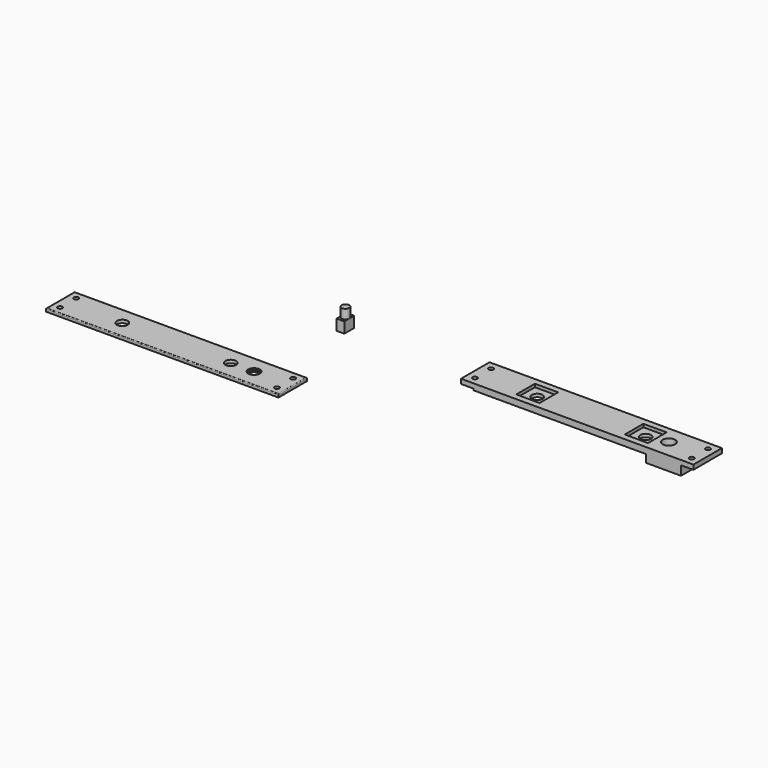
from build123d import *

# Parameters (mm, degrees)
F1_W      = 5
F1_H      = 8
F2_DEPTH  = 7
F4_DEPTH  = 6
F0_W      = 150
F0_H      = 23
F0_R      = 1.5
F0_R_2    = 3.5
F0_R_3    = 4
F5_DEPTH  = 4
F6_W      = 150
F6_H      = 23
F6_R      = 1.5
F6_R_2    = 3.5
F6_R_3    = 3.1
F7_DEPTH  = 2
F8_R      = 3.75
F9_DEPTH  = 1
F10_W     = 8
F10_H     = 1
F11_DEPTH = 30
F12_W     = 15
F12_H     = 15
F12_R     = 3.5
F13_DEPTH = 2
F14_R     = 4
F15_DEPTH = 3
F17_R     = 0.5
F16_W     = 22.5
F16_H     = 23
F16_R     = 4
F18_DEPTH = 5
F19_W     = 3
F19_H     = 7.4161984871
F20_DEPTH = 2


with BuildPart() as f2:
    # F1 (on Top) → F2 (new body)
    with BuildSketch(Plane.XY):
        with Locations((-158.8816171885, 0.1063133087)):
            Rectangle(F1_W, F1_H)
    extrude(amount=F2_DEPTH)

    # F3 (on face) → F4 (join)
    with BuildSketch(Plane.XY.offset(7)):
        with BuildLine():
            ThreePointArc((-161.3816171885, 0.1063133087), (-158.8816171885, -2.3936866913), (-156.3816171885, 0.1063133087))
            ThreePointArc((-156.3816171885, 0.1063133087), (-158.8816171885, 2.6063133087), (-161.3816171885, 0.1063133087))
        make_face()
    extrude(amount=F4_DEPTH)

    # F14 (on face) → F15 (cut)
    with BuildSketch(Plane.XY.offset(4)):
        with Locations((50, 0)):
            Circle(F14_R)
    extrude(amount=-F15_DEPTH, mode=Mode.SUBTRACT)


with BuildPart() as f5:
    # F0 (on Top) → F5 (new body)
    with BuildSketch(Plane.XY):
        Rectangle(F0_W, F0_H)
        with Locations((-70, -6.5)):
            Circle(F0_R, mode=Mode.SUBTRACT)
        with Locations((70, -6.5)):
            Circle(F0_R, mode=Mode.SUBTRACT)
        with Locations((-35, 0)):
            Circle(F0_R_2, mode=Mode.SUBTRACT)
        with Locations((-70, 6.5)):
            Circle(F0_R, mode=Mode.SUBTRACT)
        with Locations((35, 0)):
            Circle(F0_R_2, mode=Mode.SUBTRACT)
        with Locations((50, 0)):
            Circle(F0_R_3, mode=Mode.SUBTRACT)
        with Locations((70, 6.5)):
            Circle(F0_R, mode=Mode.SUBTRACT)
    extrude(amount=F5_DEPTH)

    # F10 (on face) → F11 (cut)
    with BuildSketch(Plane.XZ.offset(11.5)):
        with Locations((-71, 0.5)):
            Rectangle(F10_W, F10_H)
        with Locations((71, 0.5)):
            Rectangle(F10_W, F10_H)
    extrude(amount=-F11_DEPTH, mode=Mode.SUBTRACT)

    # F12 (on face) → F13 (cut)
    with BuildSketch(Plane.XY.offset(4)):
        with Locations((-35, 0)):
            Rectangle(F12_W, F12_H)
        with Locations((-35, 0)):
            Circle(F12_R, mode=Mode.SUBTRACT)
        with Locations((35, 0)):
            Rectangle(F12_W, F12_H)
        with Locations((35, 0)):
            Circle(F12_R, mode=Mode.SUBTRACT)
    extrude(amount=-F13_DEPTH, mode=Mode.SUBTRACT)

    # F16 (on face) → F18 (join)
    with BuildSketch(Plane.XY):
        with Locations((55.75, 0)):
            Rectangle(F16_W, F16_H)
        with Locations((50, 0)):
            Circle(F16_R, mode=Mode.SUBTRACT)
    extrude(amount=-F18_DEPTH)

    # F19 (on face) → F20 (join)
    with BuildSketch(Plane(origin=(0, 0, -5), x_dir=(1, 0, 0), z_dir=(0, 0, -1))):
        with Locations((50, 0)):
            Rectangle(F19_W, F19_H)
        with BuildLine():
            Line((48.5, 3.7080992435), (51.5, 3.7080992435))
            ThreePointArc((51.5, 3.7080992435), (50, 4), (48.5, 3.7080992435))
        make_face()
        with BuildLine():
            ThreePointArc((48.5, -3.7080992435), (50, -4), (51.5, -3.7080992435))
            Line((51.5, -3.7080992435), (48.5, -3.7080992435))
        make_face()
    extrude(amount=-F20_DEPTH)


with BuildPart() as f7:
    # F6 (on Top) → F7 (new body)
    with BuildSketch(Plane.XY):
        with Locations((-213.7417785823, -67.5485283136)):
            Rectangle(F6_W, F6_H)
        with Locations((-283.7417785823, -74.0485283136)):
            Circle(F6_R, mode=Mode.SUBTRACT)
        with Locations((-143.7417785823, -74.0485283136)):
            Circle(F6_R, mode=Mode.SUBTRACT)
        with Locations((-248.7417785823, -67.5485283136)):
            Circle(F6_R_2, mode=Mode.SUBTRACT)
        with Locations((-283.7417785823, -61.0485283136)):
            Circle(F6_R, mode=Mode.SUBTRACT)
        with Locations((-178.7417785823, -67.5485283136)):
            Circle(F6_R_2, mode=Mode.SUBTRACT)
        with Locations((-163.7417785823, -67.5485283136)):
            Circle(F6_R_3, mode=Mode.SUBTRACT)
        with Locations((-143.7417785823, -61.0485283136)):
            Circle(F6_R, mode=Mode.SUBTRACT)
    extrude(amount=F7_DEPTH)

    # F8 (on face) → F9 (cut)
    with BuildSketch(Plane.XY.offset(2)):
        with Locations((-163.7417785823, -67.5485283136)):
            Circle(F8_R)
    extrude(amount=-F9_DEPTH, mode=Mode.SUBTRACT)

    # F17
    f17_edges = [f7.edges().sort_by_distance(p)[0] for p in [
        (-288.741779, -67.548528, 2),
        (-213.741779, -56.048528, 2),
        (-213.741779, -79.048528, 2),
        (-138.741779, -67.548528, 2),
    ]]
    fillet(f17_edges, radius=F17_R)


solid = Compound([f2.part, f5.part, f7.part])
